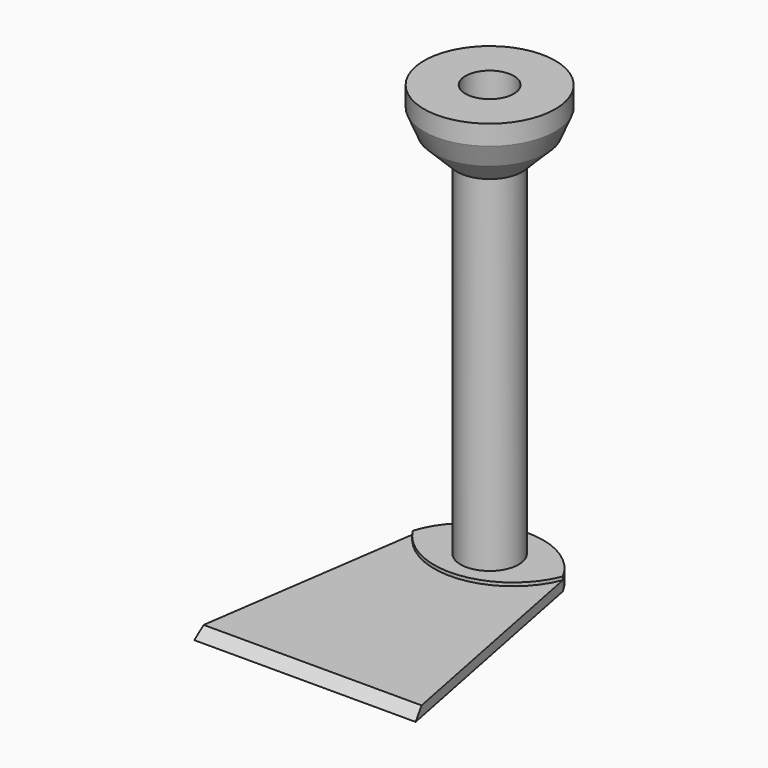
from build123d import *

# Parameters (mm, degrees)
F1_DEPTH    = 3.81
F3_T1_DEPTH = 111.8036914576
F4_DEPTH    = 1.27
F5_R        = 11.1870112164
F5_R_2      = 9.3121919152
F6_DEPTH    = 133.604
F7_R        = 25.2769928265
F7_R_2      = 11.1870112164
F7_R_3      = 9.3121919152
F8_DEPTH    = 25.4
F9_SIZE     = 12.7
F10_SIZE    = 5.08


# Not quite as in the source:
# - a fillet or chamfer that OpenCascade refuses, or shapes differently, is made with other operations: its cross-section is extruded or revolved along the edge and cut away or added


with BuildPart() as f1:
    # F0 (on Top) → F1 (new body)
    with BuildSketch(Plane.XY):
        with BuildLine():
            Line((45.1586060226, -52.2380582988), (26.3960231096, 43.0443435907))
            ThreePointArc((26.3960231096, 43.0443435907), (-2.1687844347, 58.4802777375), (-27.4601764977, 38.1194874644))
            Line((-27.4601764977, 38.1194874644), (-40.5167862773, -52.2380582988))
            Line((-40.5167862773, -52.2380582988), (45.1586060226, -52.2380582988))
        make_face()
    extrude(amount=F1_DEPTH)

    # F3: chamfer of 5.08 on 1 edges, made by hand

    # F3_s2 → F3_t1 (cut)
    with BuildSketch(Plane.YZ.offset(-53.5809358562)):
        Polygon((-52.2380582988, -1.27), (-47.1580582988, 3.81), (-52.2380582988, 3.81), align=None)
    extrude(amount=F3_T1_DEPTH, mode=Mode.SUBTRACT)

    # F2 (on face) → F4 (join)
    with BuildSketch(Plane.XY.offset(3.81)):
        with BuildLine():
            ThreePointArc((26.3960231096, 43.0443435907), (-2.1687844347, 58.4802777375), (-27.4601764977, 38.1194874644))
            ThreePointArc((-27.4601764977, 38.1194874644), (0.9757940306, 24.0924618975), (26.3960231096, 43.0443435907))
        make_face()
    extrude(amount=F4_DEPTH)

    # F5 (on face) → F6 (join)
    with BuildSketch(Plane.XY.offset(5.08)):
        with Locations((0, 40.8166870475)):
            Circle(F5_R)
        with Locations((0, 40.8166870475)):
            Circle(F5_R_2, mode=Mode.SUBTRACT)
    extrude(amount=F6_DEPTH)

    # F7 (on face) → F8 (join)
    with BuildSketch(Plane.XY.offset(138.684)):
        with Locations((0, 40.8166870475)):
            Circle(F7_R)
        with Locations((0, 40.8166870475)):
            Circle(F7_R_2, mode=Mode.SUBTRACT)
        with Locations((0, 40.8166870475)):
            Circle(F7_R_2)
        with Locations((0, 40.8166870475)):
            Circle(F7_R_3, mode=Mode.SUBTRACT)
    extrude(amount=F8_DEPTH)

    # F9
    f9_edges = [f1.edges().sort_by_distance(p)[0] for p in [
        (-25.276993, 40.816687, 138.684),
    ]]
    chamfer(f9_edges, length=F9_SIZE)

    # F10
    f10_edges = [f1.edges().sort_by_distance(p)[0] for p in [
        (-25.276993, 40.816687, 151.384),
    ]]
    chamfer(f10_edges, length=F10_SIZE)


solid = f1.part
